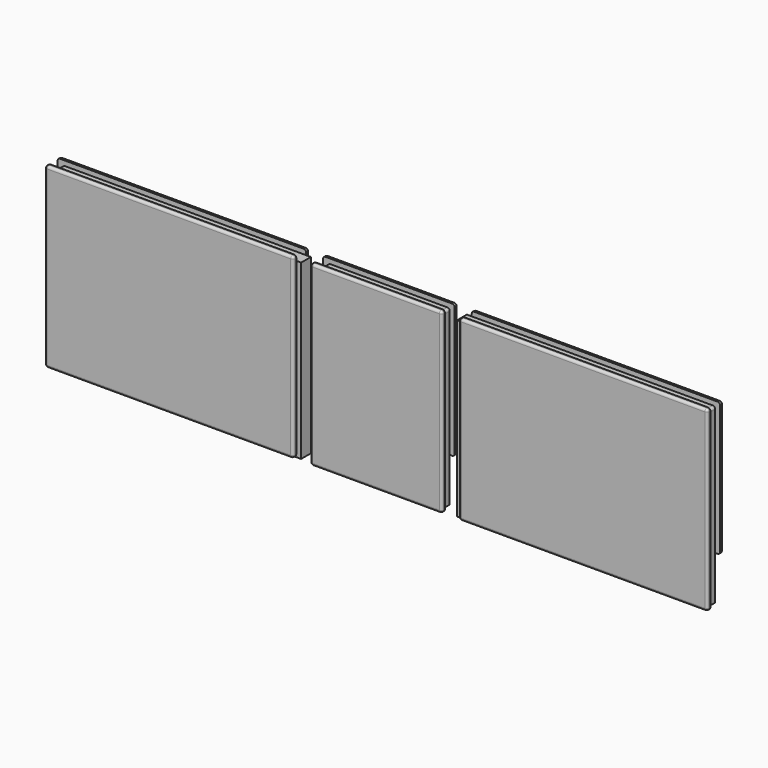
from build123d import *

# Parameters (mm, degrees)
F0_W          = 50
F0_H          = 51
F1_DEPTH      = 5
F0_H_2        = 18
F2_DEPTH      = 5
F3_W          = 50
F3_H          = 51
F4_DEPTH      = 1.6
F5_W          = 50
F5_H          = 51
F6_DEPTH      = 1.6
F7_DEPTH      = 2
F8_W          = 1.6
F8_H          = 53
F9_DEPTH      = 2
F10_W         = 1.6
F10_H         = 53
F11_DEPTH     = 2
F12_DEPTH     = 1.6
F13_DEPTH     = 18
F15_DEPTH     = 2
F16_T1_DEPTH  = 52
F16_T3_DEPTH  = 5
F16_T5_DEPTH  = 3.1
F16_T7_DEPTH  = 3.1
F16_T9_DEPTH  = 53
F16_T11_DEPTH = 71
F16_S15_W     = 1.02
F16_S15_H     = 1.02
F16_T16_DEPTH = 1.02
F16_S21_W     = 1.02
F16_S21_H     = 1.02
F16_T22_DEPTH = 1.02
F16_S27_W     = 1.02
F16_S27_H     = 1.02
F16_T28_DEPTH = 1.02
F16_S33_W     = 1.02
F16_S33_H     = 1.02
F16_T34_DEPTH = 1.02
F16_S39_W     = 1.02
F16_S39_H     = 1.02
F16_T40_DEPTH = 1.02
F16_S45_W     = 1.02
F16_S45_H     = 1.02
F16_T46_DEPTH = 1.02
F16_S51_W     = 1.02
F16_S51_H     = 1.02
F16_T52_DEPTH = 1.02
F16_S57_W     = 1.02
F16_S57_H     = 1.02
F16_T58_DEPTH = 1.02
F17_W         = 102
F17_H         = 69
F18_DEPTH     = 5
F19_W         = 100
F19_H         = 51
F20_DEPTH     = 1.6
F21_W         = 100
F21_H         = 69
F22_DEPTH     = 1.6
F23_W         = 1.6
F23_H         = 51
F23_H_2       = 69
F24_DEPTH     = 2
F25_DEPTH     = 2
F27_DEPTH     = 2
F28_R         = 1


# Not quite as in the source:
# - a fillet or chamfer that OpenCascade refuses, or shapes differently, is made with other operations: its cross-section is extruded or revolved along the edge and cut away or added


with BuildPart() as f1:
    # F0 (on Front) → F1 (new body)
    with BuildSketch(Plane.XZ):
        with Locations((0, 43.5)):
            Rectangle(F0_W, F0_H)
    extrude(amount=F1_DEPTH)

    # F0 (on Front) → F2 (join)
    with BuildSketch(Plane.XZ):
        with Locations((0, 9)):
            Rectangle(F0_W, F0_H_2)
        with Locations((0, 43.5)):
            Rectangle(F0_W, F0_H)
    extrude(amount=F2_DEPTH)

    # F3 (on face) → F4 (join)
    with BuildSketch(Plane(origin=(0, 0, 0), x_dir=(-1, 0, 0), z_dir=(0, 1, 0))):
        with Locations((0, 43.5)):
            Rectangle(F3_W, F3_H)
    extrude(amount=F4_DEPTH)

    # F5 (on face) → F6 (join)
    with BuildSketch(Plane.XZ.offset(5)):
        with Locations((0, 43.5)):
            Rectangle(F5_W, F5_H)
    extrude(amount=F6_DEPTH)

    # F7 (add): a face of the model
    f7_faces = [f1.faces().sort_by_distance(p)[0] for p in [
        (0, -2.5, 69),
    ]]
    extrude(f7_faces, amount=F7_DEPTH)

    # F8 (on face) → F9 (join)
    with BuildSketch(Plane(origin=(-25, 0, 0), x_dir=(0, -1, 0), z_dir=(-1, 0, 0))):
        with Locations((-0.8, 44.5)):
            Rectangle(F8_W, F8_H)
        with Locations((5.8, 44.5)):
            Rectangle(F8_W, F8_H)
    extrude(amount=F9_DEPTH)

    # F10 (on face) → F11 (join)
    with BuildSketch(Plane.YZ.offset(25)):
        with Locations((-5.8, 44.5)):
            Rectangle(F10_W, F10_H)
        with Locations((0.8, 44.5)):
            Rectangle(F10_W, F10_H)
    extrude(amount=F11_DEPTH)

    # F12 (add): a face of the model
    f12_faces = [f1.faces().sort_by_distance(p)[0] for p in [
        (0, -5, 9),
    ]]
    extrude(f12_faces, amount=F12_DEPTH)

    # F13 (add, through all): faces of the model
    f13_faces = [f1.faces().sort_by_distance(p)[0] for p in [
        (26, -5.8, 18),
        (-26, -5.8, 18),
    ]]
    extrude(f13_faces, amount=F13_DEPTH)

    # F14 (on face) → F15 (join)
    with BuildSketch(Plane.XY.offset(71)):
        Polygon((25, -5), (-25, -5), (-27, -5), (-27, -6.6), (27, -6.6), (27, -5), align=None)
        Polygon((-27, 0), (-25, 0), (25, 0), (27, 0), (27, 1.6), (-27, 1.6), align=None)
    extrude(amount=F15_DEPTH)

    # F16: fillet of radius 1 on 20 edges, made by hand

    # F16_s2 → F16_t1 (cut)
    with BuildSketch(Plane.YZ.offset(-26)):
        with BuildLine():
            ThreePointArc((1.6, 19), (1.3071067812, 18.2928932188), (0.6, 18))
            Line((0.6, 18), (1.6, 18))
            Line((1.6, 18), (1.6, 19))
        make_face()
        with BuildLine():
            ThreePointArc((-5.6, 0), (-6.3071067812, 0.2928932188), (-6.6, 1))
            Line((-6.6, 1), (-6.6, 0))
            Line((-6.6, 0), (-5.6, 0))
        make_face()
        with BuildLine():
            ThreePointArc((1.6, 72), (1.3071067812, 72.7071067812), (0.6, 73))
            Line((0.6, 73), (1.6, 73))
            Line((1.6, 73), (1.6, 72))
        make_face()
        with BuildLine():
            ThreePointArc((-5.6, 73), (-6.3071067812, 72.7071067812), (-6.6, 72))
            Line((-6.6, 72), (-6.6, 73))
            Line((-6.6, 73), (-5.6, 73))
        make_face()
    extrude(amount=F16_T1_DEPTH, mode=Mode.SUBTRACT)

    # F16_s4 → F16_t3 (cut)
    with BuildSketch(Plane.XZ):
        with BuildLine():
            ThreePointArc((-25, 70), (-24.7071067812, 70.7071067812), (-24, 71))
            Line((-24, 71), (-25, 71))
            Line((-25, 71), (-25, 70))
        make_face()
        with BuildLine():
            ThreePointArc((25, 70), (24.7071067812, 70.7071067812), (24, 71))
            Line((24, 71), (25, 71))
            Line((25, 71), (25, 70))
        make_face()
    extrude(amount=F16_T3_DEPTH, mode=Mode.SUBTRACT)

    # F16_s6 → F16_t5 (cut)
    with BuildSketch(Plane.XZ.offset(-0.6)):
        with BuildLine():
            ThreePointArc((-27, 19), (-26.7071067812, 18.2928932188), (-26, 18))
            Line((-26, 18), (-27, 18))
            Line((-27, 18), (-27, 19))
        make_face()
        with BuildLine():
            ThreePointArc((27, 19), (26.7071067812, 18.2928932188), (26, 18))
            Line((26, 18), (27, 18))
            Line((27, 18), (27, 19))
        make_face()
        with BuildLine():
            ThreePointArc((27, 72), (26.7071067812, 72.7071067812), (26, 73))
            Line((26, 73), (27, 73))
            Line((27, 73), (27, 72))
        make_face()
        with BuildLine():
            ThreePointArc((-26, 73), (-26.7071067812, 72.7071067812), (-27, 72))
            Line((-27, 72), (-27, 73))
            Line((-27, 73), (-26, 73))
        make_face()
    extrude(amount=F16_T5_DEPTH, mode=Mode.SUBTRACT)

    # F16_s8 → F16_t7 (cut)
    with BuildSketch(Plane.XZ.offset(2.5)):
        with BuildLine():
            ThreePointArc((27, 72), (26.7071067812, 72.7071067812), (26, 73))
            Line((26, 73), (27, 73))
            Line((27, 73), (27, 72))
        make_face()
        with BuildLine():
            ThreePointArc((-26, 73), (-26.7071067812, 72.7071067812), (-27, 72))
            Line((-27, 72), (-27, 73))
            Line((-27, 73), (-26, 73))
        make_face()
        with BuildLine():
            ThreePointArc((-26, 0), (-26.7071067812, 0.2928932188), (-27, 1))
            Line((-27, 1), (-27, 0))
            Line((-27, 0), (-26, 0))
        make_face()
        with BuildLine():
            ThreePointArc((26, 0), (26.7071067812, 0.2928932188), (27, 1))
            Line((27, 1), (27, 0))
            Line((27, 0), (26, 0))
        make_face()
    extrude(amount=F16_T7_DEPTH, mode=Mode.SUBTRACT)

    # F16_s10 → F16_t9 (cut)
    with BuildSketch(Plane.XY.offset(19)):
        with BuildLine():
            ThreePointArc((27, 0.6), (26.7071067812, 1.3071067812), (26, 1.6))
            Line((26, 1.6), (27, 1.6))
            Line((27, 1.6), (27, 0.6))
        make_face()
        with BuildLine():
            ThreePointArc((-26, 1.6), (-26.7071067812, 1.3071067812), (-27, 0.6))
            Line((-27, 0.6), (-27, 1.6))
            Line((-27, 1.6), (-26, 1.6))
        make_face()
    extrude(amount=F16_T9_DEPTH, mode=Mode.SUBTRACT)

    # F16_s12 → F16_t11 (cut)
    with BuildSketch(Plane.XY.offset(1)):
        with BuildLine():
            ThreePointArc((27, -5.6), (26.7071067812, -6.3071067812), (26, -6.6))
            Line((26, -6.6), (27, -6.6))
            Line((27, -6.6), (27, -5.6))
        make_face()
        with BuildLine():
            ThreePointArc((-26, -6.6), (-26.7071067812, -6.3071067812), (-27, -5.6))
            Line((-27, -5.6), (-27, -6.6))
            Line((-27, -6.6), (-26, -6.6))
        make_face()
    extrude(amount=F16_T11_DEPTH, mode=Mode.SUBTRACT)


with BuildPart() as f16_tool14:
    # F16_s15 → F16_t16 (new body)
    with BuildSketch(Plane.YZ.offset(26)):
        with Locations((1.11, 18.49)):
            Rectangle(F16_S15_W, F16_S15_H)
    extrude(amount=F16_T16_DEPTH)

    # F16_s17 → F16_t18 (revolve, cut)
    with BuildSketch(Plane(origin=(26, 0.6, 19), x_dir=(0, -0.7071067812, 0.7071067812), z_dir=(0, 0.7071067812, 0.7071067812))):
        with BuildLine():
            ThreePointArc((0, -1), (1, 0), (0, 1))
            Line((0, 1), (0, -1))
        make_face()
    revolve(axis=Axis((26, 0.6, 19), (1, 0, 0)), mode=Mode.SUBTRACT)


with BuildPart() as f1_1:
    add(f1.part)

    # F16_t13: cut F16_tool14
    add(f16_tool14.part, mode=Mode.SUBTRACT)


with BuildPart() as f16_tool20:
    # F16_s21 → F16_t22 (new body)
    with BuildSketch(Plane.XZ.offset(-0.6)):
        with Locations((-26.51, 18.49)):
            Rectangle(F16_S21_W, F16_S21_H)
    extrude(amount=-F16_T22_DEPTH)

    # F16_s23 → F16_t24 (revolve, cut)
    with BuildSketch(Plane(origin=(-26, 0.6, 19), x_dir=(0.7071067812, 0, 0.7071067812), z_dir=(-0.7071067812, 0, 0.7071067812))):
        with BuildLine():
            ThreePointArc((0, -1), (1, 0), (0, 1))
            Line((0, 1), (0, -1))
        make_face()
    revolve(axis=Axis((-26, 0.6, 19), (0, 1, 0)), mode=Mode.SUBTRACT)


with BuildPart() as f1_2:
    add(f1_1.part)

    # F16_t19: cut F16_tool20
    add(f16_tool20.part, mode=Mode.SUBTRACT)


with BuildPart() as f16_tool26:
    # F16_s27 → F16_t28 (new body)
    with BuildSketch(Plane.XY.offset(1)):
        with Locations((26.51, -6.11)):
            Rectangle(F16_S27_W, F16_S27_H)
    extrude(amount=-F16_T28_DEPTH)

    # F16_s29 → F16_t30 (revolve, cut)
    with BuildSketch(Plane(origin=(26, -5.6, 1), x_dir=(-0.7071067812, 0.7071067812, 0), z_dir=(-0.7071067812, -0.7071067812, 0))):
        with BuildLine():
            ThreePointArc((0, -1), (1, 0), (0, 1))
            Line((0, 1), (0, -1))
        make_face()
    revolve(axis=Axis((26, -5.6, 1), (0, 0, -1)), mode=Mode.SUBTRACT)


with BuildPart() as f1_3:
    add(f1_2.part)

    # F16_t25: cut F16_tool26
    add(f16_tool26.part, mode=Mode.SUBTRACT)


with BuildPart() as f16_tool32:
    # F16_s33 → F16_t34 (new body)
    with BuildSketch(Plane.XY.offset(1)):
        with Locations((-26.51, -6.11)):
            Rectangle(F16_S33_W, F16_S33_H)
    extrude(amount=-F16_T34_DEPTH)

    # F16_s35 → F16_t36 (revolve, cut)
    with BuildSketch(Plane(origin=(-26, -5.6, 1), x_dir=(0.7071067812, 0.7071067812, 0), z_dir=(-0.7071067812, 0.7071067812, 0))):
        with BuildLine():
            ThreePointArc((0, -1), (1, 0), (0, 1))
            Line((0, 1), (0, -1))
        make_face()
    revolve(axis=Axis((-26, -5.6, 1), (0, 0, -1)), mode=Mode.SUBTRACT)


with BuildPart() as f1_4:
    add(f1_3.part)

    # F16_t31: cut F16_tool32
    add(f16_tool32.part, mode=Mode.SUBTRACT)


with BuildPart() as f16_tool38:
    # F16_s39 → F16_t40 (new body)
    with BuildSketch(Plane.YZ.offset(26)):
        with Locations((-6.11, 72.51)):
            Rectangle(F16_S39_W, F16_S39_H)
    extrude(amount=F16_T40_DEPTH)

    # F16_s41 → F16_t42 (revolve, cut)
    with BuildSketch(Plane(origin=(26, -5.6, 72), x_dir=(0, 0.7071067812, -0.7071067812), z_dir=(0, -0.7071067812, -0.7071067812))):
        with BuildLine():
            ThreePointArc((0, -1), (1, 0), (0, 1))
            Line((0, 1), (0, -1))
        make_face()
    revolve(axis=Axis((26, -5.6, 72), (1, 0, 0)), mode=Mode.SUBTRACT)


with BuildPart() as f1_5:
    add(f1_4.part)

    # F16_t37: cut F16_tool38
    add(f16_tool38.part, mode=Mode.SUBTRACT)


with BuildPart() as f16_tool44:
    # F16_s45 → F16_t46 (new body)
    with BuildSketch(Plane.YZ.offset(26)):
        with Locations((1.11, 72.51)):
            Rectangle(F16_S45_W, F16_S45_H)
    extrude(amount=F16_T46_DEPTH)

    # F16_s47 → F16_t48 (revolve, cut)
    with BuildSketch(Plane(origin=(26, 0.6, 72), x_dir=(0, -0.7071067812, -0.7071067812), z_dir=(0, -0.7071067812, 0.7071067812))):
        with BuildLine():
            ThreePointArc((0, -1), (1, 0), (0, 1))
            Line((0, 1), (0, -1))
        make_face()
    revolve(axis=Axis((26, 0.6, 72), (1, 0, 0)), mode=Mode.SUBTRACT)


with BuildPart() as f1_6:
    add(f1_5.part)

    # F16_t43: cut F16_tool44
    add(f16_tool44.part, mode=Mode.SUBTRACT)


with BuildPart() as f16_tool50:
    # F16_s51 → F16_t52 (new body)
    with BuildSketch(Plane.XZ.offset(-0.6)):
        with Locations((-26.51, 72.51)):
            Rectangle(F16_S51_W, F16_S51_H)
    extrude(amount=-F16_T52_DEPTH)

    # F16_s53 → F16_t54 (revolve, cut)
    with BuildSketch(Plane(origin=(-26, 0.6, 72), x_dir=(0.7071067812, 0, -0.7071067812), z_dir=(0.7071067812, 0, 0.7071067812))):
        with BuildLine():
            ThreePointArc((0, -1), (1, 0), (0, 1))
            Line((0, 1), (0, -1))
        make_face()
    revolve(axis=Axis((-26, 0.6, 72), (0, 1, 0)), mode=Mode.SUBTRACT)


with BuildPart() as f1_7:
    add(f1_6.part)

    # F16_t49: cut F16_tool50
    add(f16_tool50.part, mode=Mode.SUBTRACT)


with BuildPart() as f16_tool56:
    # F16_s57 → F16_t58 (new body)
    with BuildSketch(Plane.XY.offset(72)):
        with Locations((-26.51, -6.11)):
            Rectangle(F16_S57_W, F16_S57_H)
    extrude(amount=F16_T58_DEPTH)

    # F16_s59 → F16_t60 (revolve, cut)
    with BuildSketch(Plane(origin=(-26, -5.6, 72), x_dir=(0.7071067812, 0.7071067812, 0), z_dir=(0.7071067812, -0.7071067812, 0))):
        with BuildLine():
            ThreePointArc((0, -1), (1, 0), (0, 1))
            Line((0, 1), (0, -1))
        make_face()
    revolve(axis=Axis((-26, -5.6, 72), (0, 0, 1)), mode=Mode.SUBTRACT)


with BuildPart() as f1_8:
    add(f1_7.part)

    # F16_t55: cut F16_tool56
    add(f16_tool56.part, mode=Mode.SUBTRACT)


with BuildPart() as f18:
    # F17 (on Front) → F18 (new body)
    with BuildSketch(Plane.XZ):
        with Locations((83.031789422, 34.5)):
            Rectangle(F17_W, F17_H)
    extrude(amount=F18_DEPTH)

    # F19 (on face) → F20 (join)
    with BuildSketch(Plane(origin=(0, 0, 0), x_dir=(-1, 0, 0), z_dir=(0, 1, 0))):
        with Locations((-84.031789422, 43.5)):
            Rectangle(F19_W, F19_H)
    extrude(amount=F20_DEPTH)

    # F21 (on face) → F22 (join)
    with BuildSketch(Plane.XZ.offset(5)):
        with Locations((84.031789422, 34.5)):
            Rectangle(F21_W, F21_H)
    extrude(amount=F22_DEPTH)

    # F23 (on face) → F24 (join)
    with BuildSketch(Plane.YZ.offset(134.031789422)):
        with Locations((0.8, 43.5)):
            Rectangle(F23_W, F23_H)
        with Locations((-5.8, 34.5)):
            Rectangle(F23_W, F23_H_2)
    extrude(amount=F24_DEPTH)

    # F25 (add): a face of the model
    f25_faces = [f18.faces().sort_by_distance(p)[0] for p in [
        (83.8122772269, -2.5, 69),
    ]]
    extrude(f25_faces, amount=F25_DEPTH)

    # F26 (on face) → F27 (join)
    with BuildSketch(Plane.XY.offset(71)):
        Polygon((136.031789422, -5), (134.031789422, -5), (34.031789422, -5), (34.031789422, -6.6), (136.031789422, -6.6), align=None)
        Polygon((34.031789422, 1.6), (34.031789422, 0), (134.031789422, 0), (136.031789422, 0), (136.031789422, 1.6), align=None)
    extrude(amount=F27_DEPTH)

    # F28
    f28_edges = [f18.edges().sort_by_distance(p)[0] for p in [
        (34.031789, -6.6, 36.5),
        (85.031789, -6.6, 0),
        (136.031789, -6.6, 36.5),
        (85.031789, -6.6, 73),
        (34.031789, -5.8, 0),
        (136.031789, 1.6, 45.5),
        (85.031789, 1.6, 73),
        (34.031789, 1.6, 45.5),
        (85.031789, 1.6, 18),
        (34.031789, 0.8, 18),
        (134.031789, -2.5, 71),
        (34.031789, -5.8, 73),
        (136.031789, -5.8, 73),
        (136.031789, -5.8, 0),
        (136.031789, 0.8, 18),
        (136.031789, 0.8, 73),
        (34.031789, 0.8, 73),
    ]]
    fillet(f28_edges, radius=F28_R)


with BuildPart() as f29_1:
    # F29: instance of F18
    add(f18.part.mirror(Plane.YZ))


solid = Compound([f1_8.part, f18.part, f29_1.part])
